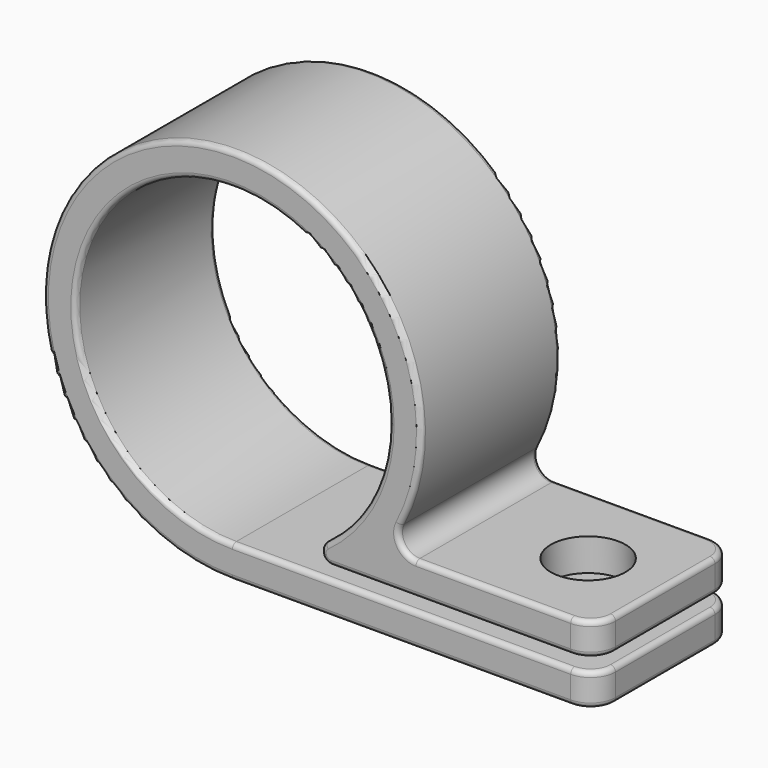
from build123d import *

# Parameters (mm, degrees)
F1_DEPTH = 7
F2_R     = 2
F3_R     = 1.4
F4_R     = 0.8
F6_DEPTH = 6.201
F7_R     = 0.4


with BuildPart() as f1:
    # F0 (on Front) → F1 (new body, symmetric)
    with BuildSketch(Plane.XZ):
        with BuildLine():
            ThreePointArc((0, -12.6), (-8.909545, 8.909545), (12.6, 0))
            ThreePointArc((12.6, 0), (10.505803, -6.956155), (4.91935, -11.6))
            Line((4.91935, -11.6), (29.2, -11.6))
            Line((29.2, -11.6), (29.2, -9))
            Line((29.2, -9), (12.249082, -9))
            ThreePointArc((12.249082, -9), (-6.864401, 13.561711), (0, -15.2))
            Line((0, -15.2), (29.2, -15.2))
            Line((29.2, -15.2), (29.2, -12.6))
            Line((29.2, -12.6), (0, -12.6))
        make_face()
    extrude(amount=F1_DEPTH, both=True)

    # F2
    f2_edges = [f1.edges().sort_by_distance(p)[0] for p in [
        (29.2, -7, -10.3),
        (29.2, -7, -13.9),
        (29.2, 7, -13.9),
        (29.2, 7, -10.3),
    ]]
    fillet(f2_edges, radius=F2_R)

    # F3
    f3_edges = [f1.edges().sort_by_distance(p)[0] for p in [
        (12.249082, 3.5, -9),
        (12.249082, -3.5, -9),
    ]]
    fillet(f3_edges, radius=F3_R)

    # F4
    f4_edges = [f1.edges().sort_by_distance(p)[0] for p in [
        (4.91935, 3.5, -11.6),
        (4.91935, -3.5, -11.6),
    ]]
    fillet(f4_edges, radius=F4_R)

    # F5 (on face) → F6 (cut, through all)
    with BuildSketch(Plane.XY.offset(-9)):
        with BuildLine():
            Line((20, 0), (26, 0))
            ThreePointArc((26, 0), (23, 3), (20, 0))
        make_face()
        with BuildLine():
            ThreePointArc((20, 0), (23, -3), (26, 0))
            Line((26, 0), (20, 0))
        make_face()
    extrude(amount=-F6_DEPTH, mode=Mode.SUBTRACT)

    # F7
    f7_edges = [f1.edges().sort_by_distance(p)[0] for p in [
        (-7.913996, -7, 12.977237),
        (-3.92455, -7, 11.973216),
    ]]
    fillet(f7_edges, radius=F7_R)


solid = f1.part
